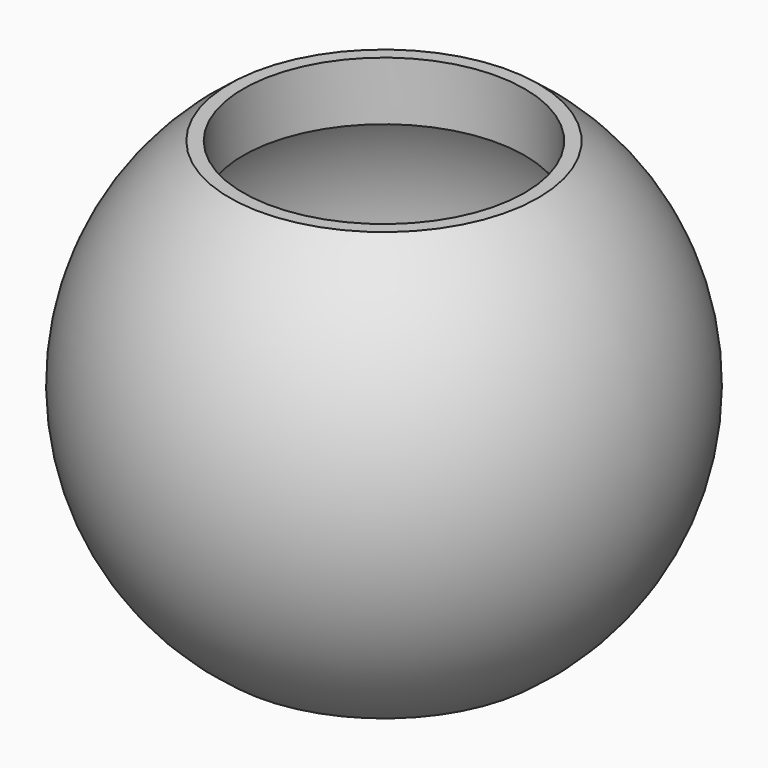
from build123d import *

# Parameters (mm, degrees)
F2_R          = 60.96
F3_DEPTH      = 114.301
F3_DEPTH_BACK = 114.301
F4_W          = 259.588
F4_H          = 37.084
F5_DEPTH      = 114.301
F5_DEPTH_BACK = 114.301


with BuildPart() as f1:
    # F0 (on Front) → F1 (revolve)
    with BuildSketch(Plane.XZ):
        with BuildLine():
            Line((0, 114.3), (0, -114.3))
            ThreePointArc((0, -114.3), (114.3, 0), (0, 114.3))
        make_face()
    revolve(axis=Axis((0, 0, 0), (0, 0, -1)))

    # F2 (on Top) → F3 (cut, two sides)
    with BuildSketch(Plane.XY) as f3_sk:
        Circle(F2_R)
    extrude(amount=-F3_DEPTH, mode=Mode.SUBTRACT)
    extrude(f3_sk.sketch, amount=F3_DEPTH_BACK, mode=Mode.SUBTRACT)

    # F4 (on Front) → F5 (cut, two sides)
    with BuildSketch(Plane.XZ) as f5_sk:
        with Locations((0, 111.252)):
            Rectangle(F4_W, F4_H)
        with Locations((0, -111.252)):
            Rectangle(F4_W, F4_H)
    extrude(amount=-F5_DEPTH, mode=Mode.SUBTRACT)
    extrude(f5_sk.sketch, amount=F5_DEPTH_BACK, mode=Mode.SUBTRACT)

    # F6 (on Right) → F7 (revolve, cut)
    with BuildSketch(Plane.YZ):
        with BuildLine():
            Line((0, 67.31), (-76.1046903942, 67.31))
            ThreePointArc((-76.1046903942, 67.31), (-101.6, 0), (-76.1046903942, -67.31))
            Line((-76.1046903942, -67.31), (0, -67.31))
            Line((0, -67.31), (0, 67.31))
        make_face()
    revolve(axis=Axis((0, 0, 0), (0, 0, 1)), mode=Mode.SUBTRACT)


solid = f1.part
